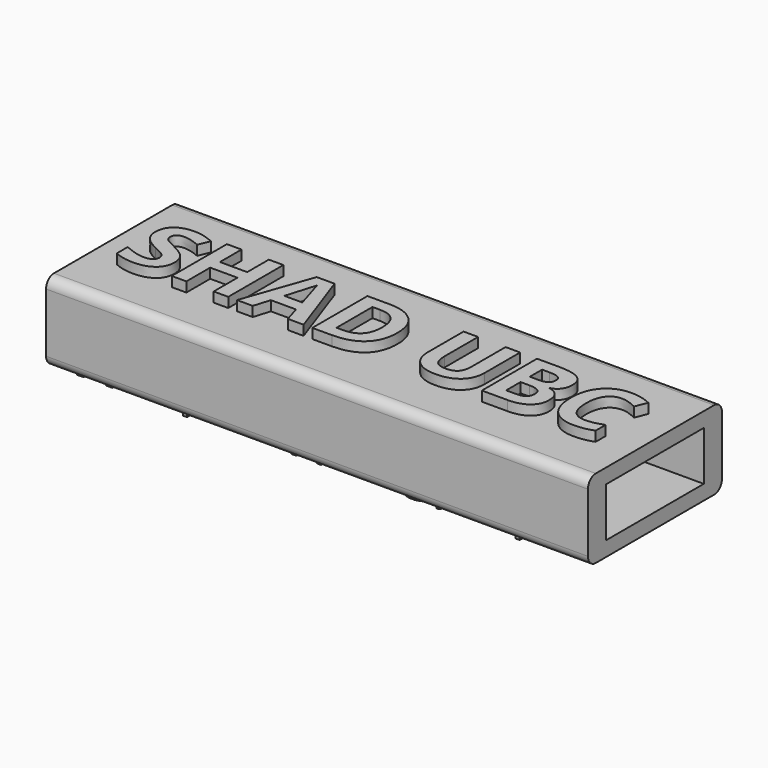
from build123d import *

# Parameters (mm, degrees)
F1_DEPTH     = 27.5
F2_W         = 12.4
F2_H         = 5
F3_DEPTH     = 14
F4_ANGLE     = -90
F6_TEXT_SIZE = 9.8024199724
F7_DEPTH     = 1
F8_TEXT_SIZE = 5.0912584054
F10_DEPTH    = 1
F9_TEXT_SIZE = 9.4981111711
F11_DEPTH    = 1


# Not quite as in the source:
# - Text() gives the source's letters only with a copy of the font that has no kerning and outlines rounded to 1/6400 em; it was checked with that copy


with BuildPart() as f1:
    # F0 (on Front) → F1 (new body, symmetric)
    with BuildSketch(Plane.XZ):
        with BuildLine():
            Line((7.5, 4), (-7.5, 4))
            ThreePointArc((-7.5, 4), (-8.2071067812, 3.7071067812), (-8.5, 3))
            Line((-8.5, 3), (-8.5, -3))
            ThreePointArc((-8.5, -3), (-8.2071067812, -3.7071067812), (-7.5, -4))
            Line((-7.5, -4), (7.5, -4))
            ThreePointArc((7.5, -4), (8.2071067812, -3.7071067812), (8.5, -3))
            Line((8.5, -3), (8.5, 3))
            ThreePointArc((8.5, 3), (8.2071067812, 3.7071067812), (7.5, 4))
        make_face()
    extrude(amount=F1_DEPTH, both=True)

    # F2 (on face) → F3 (cut)
    with BuildSketch(Plane.XZ.offset(27.5)):
        Rectangle(F2_W, F2_H)
    extrude(amount=-F3_DEPTH, mode=Mode.SUBTRACT)


with BuildPart() as f1_1:
    # F4: moved
    add(f1.part.rotate(Axis((8.5, 27.5, 0), (0, 0, -1)), F4_ANGLE))


with BuildPart() as f1_2:
    # F5: moved
    add(f1_1.part.moved(Location((-36, -19, 0))))

    # F6 (on face) → F7 (join)
    with BuildSketch(Plane.XY.offset(4)):
        with Locations((-25, -3.5288723802)):
            Text('SHAD UBC', F6_TEXT_SIZE, font='Open Sans', font_style=FontStyle.BOLD, text_align=(TextAlign.LEFT, TextAlign.BOTTOM))
    extrude(amount=F7_DEPTH)

    # F8 (on face) → F10 (join)
    with BuildSketch(Plane(origin=(0, 0, -4), x_dir=(1, 0, 0), z_dir=(0, 0, -1))):
        with Locations((-26.5, 2.8342939481)):
            Text('Matthew Van Oirschot', F8_TEXT_SIZE, font='Open Sans', text_align=(TextAlign.LEFT, TextAlign.BOTTOM))
    extrude(amount=F10_DEPTH)

    # F9 (on face) → F11 (join)
    with BuildSketch(Plane(origin=(0, 0, -4), x_dir=(1, 0, 0), z_dir=(0, 0, -1))):
        with Locations((-11, -6.5000000432)):
            Text('2017', F9_TEXT_SIZE, font='Open Sans', font_style=FontStyle.BOLD, text_align=(TextAlign.LEFT, TextAlign.BOTTOM))
    extrude(amount=F11_DEPTH)


solid = f1_2.part
